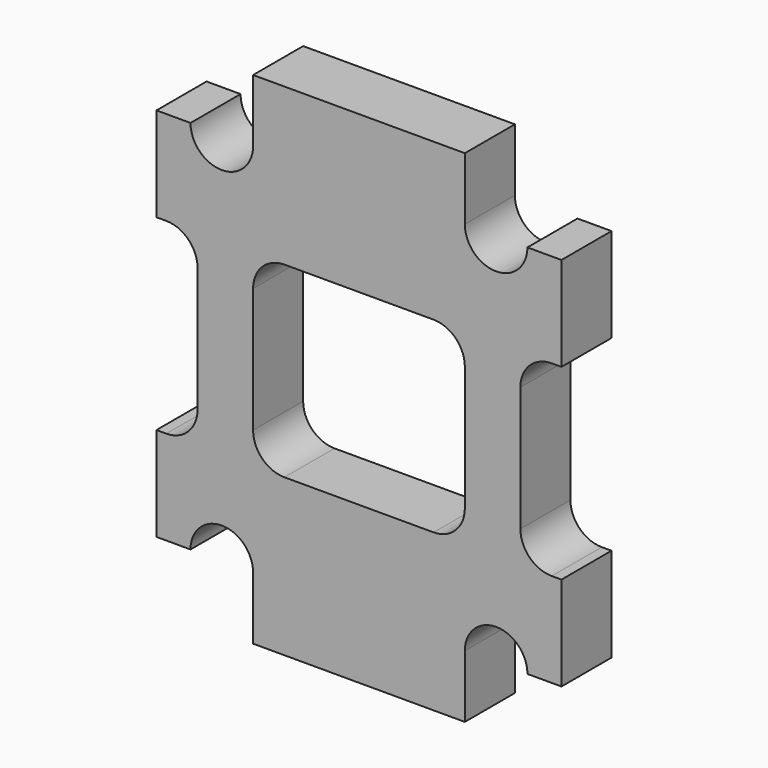
from build123d import *

# Parameters (mm, degrees)
F1_DEPTH = 6.35


# Not quite as in the source:
# - ends of sketch curves that miss each other by under 0.0002 mm in the source are joined


with BuildPart() as f1:
    # F0 (on Front) → F1 (new body)
    with BuildSketch(Plane.XZ):
        with BuildLine():
            ThreePointArc((10.7423712, -19.0500001571), (13.9173712, -15.8750001571), (17.0923712, -19.0500001571))
            Line((17.0923712, -19.0500001571), (20.545679, -19.0500001571))
            Line((20.545679, -19.0500001571), (20.545679, -9.4996001571))
            Line((20.545679, -9.4996001571), (19.5523612, -9.4996001571))
            ThreePointArc((19.5523612, -9.4996001571), (17.3072971697, -8.5696641874), (16.3773612, -6.3246001571))
            Line((16.3773612, -6.3246001571), (16.3773612, 6.3245998429))
            ThreePointArc((16.3773612, 6.3245998429), (17.3072971697, 8.5696638731), (19.5523612, 9.4995998429))
            Line((19.5523612, 9.4995998429), (20.545679, 9.4995998429))
            Line((20.545679, 9.4995998429), (20.545679, 19.0499998429))
            Line((20.545679, 19.0499998429), (17.0923712, 19.0499998429))
            ThreePointArc((17.0923712, 19.0499998429), (13.9173712, 15.8749998429), (10.7423712, 19.0499998429))
            Line((10.7423712, 19.0499998429), (10.7423712, 25.3999998429))
            Line((10.7423712, 25.3999998429), (-10.7423712, 25.3999998429))
            Line((-10.7423712, 25.3999998429), (-10.7423712, 19.0499998429))
            ThreePointArc((-10.7423712, 19.0499998429), (-13.9173712, 15.8749998429), (-17.0923712, 19.0499998429))
            Line((-17.0923712, 19.0499998429), (-20.545679, 19.0499998429))
            Line((-20.545679, 19.0499998429), (-20.545679, 9.4995998429))
            Line((-20.545679, 9.4995998429), (-19.5523612, 9.4995998429))
            ThreePointArc((-19.5523612, 9.4995998429), (-17.3072971697, 8.5696638731), (-16.3773612, 6.3245998429))
            Line((-16.3773612, 6.3245998429), (-16.3773612, -6.3246001571))
            ThreePointArc((-16.3773612, -6.3246001571), (-17.3072971697, -8.5696641874), (-19.5523612, -9.4996001571))
            Line((-19.5523612, -9.4996001571), (-20.545679, -9.4996001571))
            Line((-20.545679, -9.4996001571), (-20.545679, -19.0500001571))
            Line((-20.545679, -19.0500001571), (-17.0923712, -19.0500001571))
            ThreePointArc((-17.0923712, -19.0500001571), (-13.9173712, -15.8750001571), (-10.7423712, -19.0500001571))
            Line((-10.7423712, -19.0500001571), (-10.7423712, -25.3999747571))
            Line((-10.7423712, -25.3999747571), (10.7423712, -25.3999747571))
            Line((10.7423712, -25.3999747571), (10.7423712, -19.0500001571))
        make_face()
        with BuildLine():
            Line((-7.5673712, 9.4996252429), (7.5673712, 9.4996252429))
            ThreePointArc((7.5673712, 9.4996252429), (9.8124352303, 8.5696638731), (10.7423712, 6.3245998429))
            Line((10.7423712, 6.3245998429), (10.7423712, -6.3246001571))
            ThreePointArc((10.7423712, -6.3246001571), (9.8124352303, -8.5696641874), (7.5673712, -9.4996001571))
            Line((7.5673712, -9.4996001571), (-7.5673712, -9.4996001571))
            ThreePointArc((-7.5673712, -9.4996001571), (-9.8124352303, -8.5696641874), (-10.7423712, -6.3246001571))
            Line((-10.7423712, -6.3246001571), (-10.7423712, 6.3245998429))
            ThreePointArc((-10.7423712, 6.3245998429), (-9.8124352303, 8.5696638731), (-7.5673712, 9.4996252429))
        make_face(mode=Mode.SUBTRACT)
    extrude(amount=F1_DEPTH)


solid = f1.part
